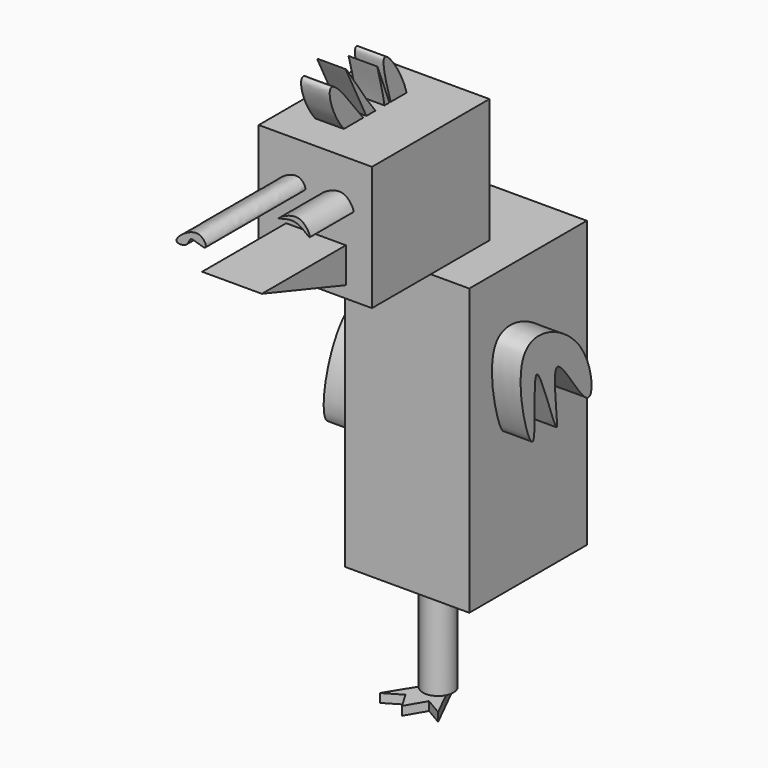
from build123d import *

# Parameters (mm, degrees)
F0_W      = 29.9761854112
F0_H      = 58.2792051136
F1_DEPTH  = 25.4
F2_R      = 3.1106368609
F3_DEPTH  = 25.4
F5_DEPTH  = 1.778
F7_DEPTH  = 7.62
F10_W     = 17.5181124359
F10_H     = 14.9880927056
F11_DEPTH = 25.4
F13_DEPTH = 12.192
F15_DEPTH = 11.176
F17_DEPTH = 25.4
F19_DEPTH = 5.842
F22_DEPTH = 5.842


# Not quite as in the source:
# - the program builds the solid bodies; features that only make, move or delete a surface that nothing else refers to are left out


with BuildPart() as f1:
    # F0 (on Right) → F1 (new body)
    with BuildSketch(Plane.YZ):
        Rectangle(F0_W, F0_H)
    extrude(amount=F1_DEPTH)

    # F2 (on face) → F3 (join)
    with BuildSketch(Plane(origin=(0, 0, -29.1396025568), x_dir=(1, 0, 0), z_dir=(0, 0, -1))):
        with Locations((7.0494809188, 0)):
            Circle(F2_R)
    extrude(amount=F3_DEPTH)

    # F4 (on face) → F5 (join)
    with BuildSketch(Plane(origin=(0, 0, -54.5396025568), x_dir=(1, 0, 0), z_dir=(0, 0, -1))):
        with BuildLine():
            Line((4.5352468525, 1.8315809401), (7.5484365778, -3.0703590882))
            Line((7.5484365778, -3.0703590882), (9.8016124347, 1.4497702575))
            ThreePointArc((9.8016124347, 1.4497702575), (7.2744112379, 3.1024938407), (4.5352468525, 1.8315809401))
        make_face()
        with BuildLine():
            ThreePointArc((4.5352468525, 1.8315809401), (7.2744112379, 3.1024938407), (9.8016124347, 1.4497702575))
            Line((9.8016124347, 1.4497702575), (12.4411685392, 6.7450227216))
            Line((12.4411685392, 6.7450227216), (8.9516591602, 4.7101395455))
            Line((8.9516591602, 4.7101395455), (6.6280206473, 8.6948195899))
            Line((6.6280206473, 8.6948195899), (4.6368231997, 5.3251436912))
            Line((4.6368231997, 5.3251436912), (1.1048497138, 7.4122454782))
            Line((1.1048497138, 7.4122454782), (4.5352468525, 1.8315809401))
        make_face()
    extrude(amount=F5_DEPTH)

    # F6 (on face) → F7 (join)
    with BuildSketch(Plane(origin=(0, 0, 0), x_dir=(0, -1, 0), z_dir=(-1, 0, 0))):
        with BuildLine():
            add(Edge.make_bspline(
                [(4.7123748809, 10.5073554441), (10.4020048834, 6.0469216692), (14.482753043, -18.4096027525), (-5.924829801, 9.2176141253), (10.0042769088, -19.2015895825), (-6.0488841899, 0.9479463993), (1.6722222045, -22.7808454121), (-17.4173194452, 7.1929346827), (-0.4690624248, 14.5693872372), (4.7123748809, 10.5073554441)],
                knots=[0, 0, 0, 0, 0.1702154393, 0.3068048429, 0.4434138565, 0.5613719669, 0.6725211035, 0.8449880525, 1, 1, 1, 1], degree=3))
        make_face()
    extrude(amount=F7_DEPTH)

    # F10 (on face) → F11 (join)
    with BuildSketch(Plane.XY.offset(29.1396025568)):
        Polygon((0, -14.9880927056), (0, 0), (-5.5969236419, 0), (-5.5969236419, -29.9761854112), (17.5181124359, -29.9761854112), (17.5181124359, -14.9880927056), align=None)
        with Locations((8.759056218, -7.4940463528)):
            Rectangle(F10_W, F10_H)
    extrude(amount=F11_DEPTH)

    # F12 (on Right) → F13 (join)
    with BuildSketch(Plane.YZ):
        Polygon((-22.8722672909, 29.1646625847), (-20.4338971525, 38.709346205), (-51.4278113842, 38.709346205), align=None)
    extrude(amount=F13_DEPTH)

    # F14 (on face) → F15 (join)
    with BuildSketch(Plane.XZ.offset(29.9761854112)):
        with BuildLine():
            add(Edge.make_bspline(
                [(7.3997783475, 46.5327911079), (7.4300555129, 46.726396017), (12.017649382, 49.7361544129), (14.8446983557, 43.366029917), (11.067123155, 48.2044418567), (7.3730806541, 46.3620748461), (7.3997783475, 46.5327911079)],
                knots=[0, 0, 0, 0, 0.2723163892, 0.5159372032, 0.7598778037, 1, 1, 1, 1], degree=3))
        make_face()
    extrude(amount=F15_DEPTH)

    # F16 (on face) → F17 (join)
    with BuildSketch(Plane.XZ.offset(29.9761854112)):
        with BuildLine():
            add(Edge.make_bspline(
                [(-2.0670865197, 45.1764985919), (-2.2679260704, 45.9720796488), (2.5215394339, 49.7424392175), (4.9757332108, 44.6433833293), (0.3954107527, 47.3683932594), (0.5841652854, 44.8038853937), (-1.9397473834, 44.6720730229), (-2.0670865197, 45.1764985919)],
                knots=[0, 0, 0, 0, 0.2750710154, 0.4661163886, 0.6725564717, 0.8255955791, 1, 1, 1, 1], degree=3))
        make_face()
    extrude(amount=F17_DEPTH)

    # F18 (on Right) → F19 (join)
    with BuildSketch(Plane.YZ):
        with BuildLine():
            add(Edge.make_bspline(
                [(-6.3446098939, 51.6193211079), (-5.4686944606, 55.6666483448), (-16.9306163999, 72.6376345133), (-6.0774124126, 41.5001725985), (-17.3834556406, 71.8842029817), (-7.5174079129, 41.9776794539), (-28.9896907381, 76.9763396034), (-9.9984881416, 42.8537482337), (-29.247075277, 71.4973178557), (-23.5677841822, 49.2150494774), (-7.2855115917, 47.2717129661), (-6.3446098939, 51.6193211079)],
                knots=[0, 0, 0, 0, 0.1127567676, 0.2194518366, 0.3249883567, 0.4223014786, 0.5462414706, 0.6595249944, 0.7745385529, 0.8788775377, 1, 1, 1, 1], degree=3))
        make_face()
    extrude(amount=F19_DEPTH)

    # F21 (on face) → F22 (join)
    with BuildSketch(Plane.YZ.offset(25.4)):
        with BuildLine():
            add(Edge.make_bspline(
                [(6.1302091926, 11.8981283158), (9.2829648971, 7.4126280593), (10.0014106037, -5.123945743), (-3.0801152221, 20.0223455827), (2.4864670128, -10.6633195664), (-7.1674971904, 22.6973479765), (-3.9501833723, -11.8007639922), (-14.4813659577, 23.9681879448), (2.2334347969, 17.4421615965), (6.1302091926, 11.8981283158)],
                knots=[0, 0, 0, 0, 0.1272698868, 0.264929306, 0.3972562607, 0.5409842834, 0.6787999232, 0.8426956978, 1, 1, 1, 1], degree=3))
        make_face()
    extrude(amount=F22_DEPTH)


solid = f1.part
